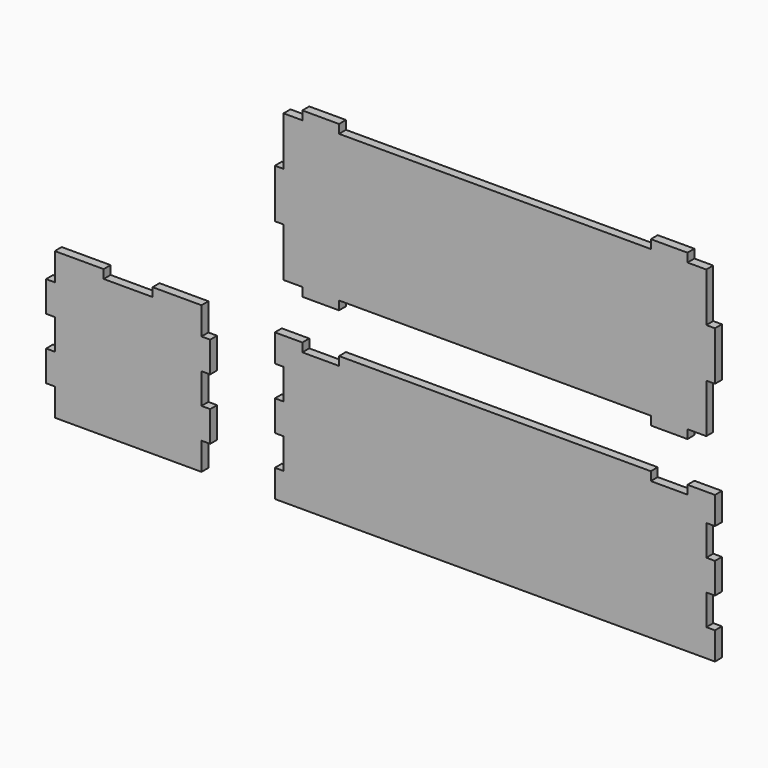
from build123d import *

# Parameters (mm, degrees)
F1_W     = 18.034
F1_H     = 63.5
F2_DEPTH = 18.034
F1_W_2   = 76.2
F1_H_2   = 18.034
F1_H_3   = 101.6


# Not quite as in the source:
# - a variable given as a bare number and used for a length is read in inches; the dataset says mm whatever the document's units were


with BuildPart() as f2:
    # F1 (on Front) → F2 (new body)
    with BuildSketch(Plane.XZ):
        Polygon((-609.6, 95.25), (-609.6, 152.4), (-711.2, 152.4), (-711.2, 134.366), (-812.8, 134.366), (-812.8, 152.4), (-914.4, 152.4), (-914.4, 95.25), (-914.4, 31.75), (-914.4, -31.75), (-914.4, -95.25), (-914.4, -152.4), (-609.6, -152.4), (-609.6, -95.25), (-609.6, -31.75), (-609.6, 31.75), align=None)
        with Locations((-923.417, 63.5)):
            Rectangle(F1_W, F1_H)
        with Locations((-923.417, -63.5)):
            Rectangle(F1_W, F1_H)
        with Locations((-600.583, 63.5)):
            Rectangle(F1_W, F1_H)
        with Locations((-600.583, -63.5)):
            Rectangle(F1_W, F1_H)
    extrude(amount=F2_DEPTH)


with BuildPart() as f2b:
    # F1 (on Front) → F2, piece 2 (new body)
    with BuildSketch(Plane.XZ):
        Polygon((-400.05, 152.4), (-457.2, 152.4), (-457.2, 95.25), (-439.166, 95.25), (-439.166, 31.75), (-457.2, 31.75), (-457.2, -31.75), (-439.166, -31.75), (-439.166, -95.25), (-457.2, -95.25), (-457.2, -152.4), (457.2, -152.4), (457.2, -95.25), (439.166, -95.25), (439.166, -31.75), (457.2, -31.75), (457.2, 31.75), (439.166, 31.75), (439.166, 95.25), (457.2, 95.25), (457.2, 152.4), (400.05, 152.4), (400.05, 134.366), (323.85, 134.366), (323.85, 152.4), (-323.85, 152.4), (-323.85, 134.366), (-400.05, 134.366), align=None)
    extrude(amount=F2_DEPTH)


with BuildPart() as f2c:
    # F1 (on Front) → F2, piece 3 (new body)
    with BuildSketch(Plane.XZ):
        Polygon((-439.166, 254), (-400.05, 254), (-323.85, 254), (323.85, 254), (400.05, 254), (439.166, 254), (439.166, 355.6), (439.166, 457.2), (439.166, 558.8), (400.05, 558.8), (323.85, 558.8), (-323.85, 558.8), (-400.05, 558.8), (-439.166, 558.8), (-439.166, 457.2), (-439.166, 355.6), align=None)
        with Locations((-361.95, 567.817)):
            Rectangle(F1_W_2, F1_H_2)
        with Locations((361.95, 567.817)):
            Rectangle(F1_W_2, F1_H_2)
        with Locations((361.95, 244.983)):
            Rectangle(F1_W_2, F1_H_2)
        with Locations((-361.95, 244.983)):
            Rectangle(F1_W_2, F1_H_2)
        with Locations((-448.183, 406.4)):
            Rectangle(F1_W, F1_H_3)
        with Locations((448.183, 406.4)):
            Rectangle(F1_W, F1_H_3)
    extrude(amount=F2_DEPTH)


solid = Compound([f2.part, f2b.part, f2c.part])
